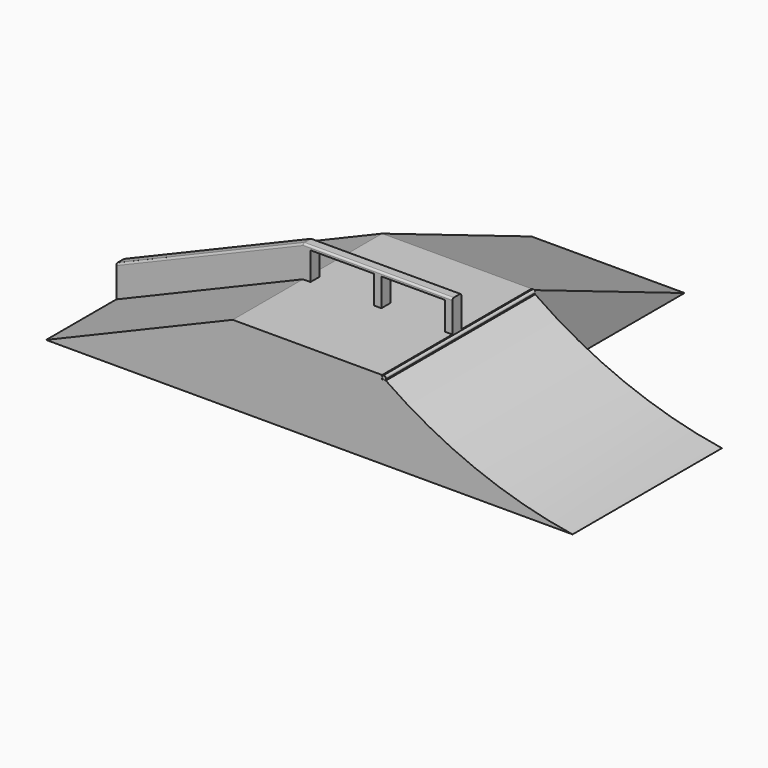
from build123d import *

# Parameters (mm, degrees)
F1_DEPTH     = 127
F2_W         = 5.08
F2_H         = 7.62
F3_DEPTH     = 19.05
F4_W         = 7.62
F4_H         = 2.54
F5_DEPTH     = 101.6
F6_T         = 5.08
F6_T3_DEPTH  = 17.78
F6_T5_DEPTH  = 15.24
F6_T7_DEPTH  = 15.24
F6_T9_DEPTH  = 15.24
F6_T11_DEPTH = 137.16
F8_DEPTH     = 7.62
F10_DEPTH    = 104.14
F11_R        = 1.27


# Not quite as in the source:
# - a shell that OpenCascade refuses in one call is made with other operations: the cavity is built on its own and cut out
# - a feature names something its author has since deleted; it is built from what else it names


with BuildPart() as f1:
    # F0 (on Front) → F1 (new body)
    with BuildSketch(Plane.XZ):
        with BuildLine():
            Line((0, 50.8), (0, 0))
            Line((0, 0), (127, 0))
            ThreePointArc((127, 0), (60.6135499229, 18.1838748072), (0, 50.8))
        make_face()
        Polygon((-104.14, 0), (-2.54, 0), (-2.54, 50.8), (-2.54, 52.07), (-2.54, 53.34), (-104.14, 53.34), align=None)
        Polygon((-2.54, 0), (0, 0), (0, 50.8), (-1.27, 50.8), (-2.54, 50.8), align=None)
        Polygon((-231.14, 0), (-104.14, 0), (-104.14, 53.34), align=None)
    extrude(amount=F1_DEPTH)

    # F2 (on face) → F3 (join)
    with BuildSketch(Plane.XY.offset(53.34)):
        with Locations((-101.6, -63.5)):
            Rectangle(F2_W, F2_H)
        with Locations((-5.08, -63.5)):
            Rectangle(F2_W, F2_H)
        with Locations((-53.34, -63.5)):
            Rectangle(F2_W, F2_H)
    extrude(amount=F3_DEPTH)

    # F4 (on face) → F5 (join)
    with BuildSketch(Plane.YZ.offset(-2.54)):
        with Locations((-63.5, 73.66)):
            Rectangle(F4_W, F4_H)
    extrude(amount=-F5_DEPTH)

    # F6: shell of thickness 5.08, made by hand


with BuildPart() as f1b:
    # F0 (on Front) → F1, piece 2 (new body)
    with BuildSketch(Plane.XZ):
        with BuildLine():
            ThreePointArc((-2.54, 52.07), (-2.1680256121, 51.1719743879), (-1.27, 50.8))
            ThreePointArc((-1.27, 50.8), (-0.3719743879, 51.1719743879), (0, 52.07))
            ThreePointArc((0, 52.07), (-1.27, 53.34), (-2.54, 52.07))
        make_face()
    extrude(amount=F1_DEPTH)


with BuildPart() as f6_core1:
    # F6_t2: copy of F1
    add(f1.part)

    # the walls: a layer under each face that stays
    f6_faces = [f6_core1.faces().sort_by_distance(p)[0] for p in [
        (60.6135499229, -63.5, 18.1838748072),
        (-52.07, -127, 26.67),
        (-167.64, -63.5, 26.67),
        (-104.14, -63.5, 64.135),
        (-53.34, -67.31, 64.135),
        (-99.06, -63.5, 62.865),
        (-77.47, -63.5, 72.39),
        (-55.88, -63.5, 62.865),
        (-50.8, -63.5, 62.865),
        (-29.21, -63.5, 72.39),
        (-7.62, -63.5, 62.865),
        (-53.34, -63.5, 74.93),
        (-53.34, -59.69, 64.135),
        (-19.4733333333, -105.8333333333, 53.34),
        (-2.54, -63.5, 62.865),
        (-52.07, 0, 26.67),
        (-1.27, -63.5, 50.8),
    ]]
    thicken(f6_faces, amount=-F6_T, mode=Mode.SUBTRACT)

    # F6_s4 → F6_t3 (cut)
    with BuildSketch(Plane.XZ.offset(54.61)):
        Polygon((-104.2104714102, 53.386836691), (-102.1728589795, 48.6563309035), (-99.06, 49.9637316749), (-99.06, 53.34), align=None)
        Polygon((-99.0092, 53.3908), (-104.14, 53.34), (-104.14, 48.26), (-99.06, 48.26), align=None)
        Polygon((-99.0092, 72.3392), (-104.14, 72.39), (-104.14, 77.47), (-99.06, 77.47), align=None)
        Polygon((-55.9308, 72.3392), (-55.88, 77.47), (-50.8, 77.47), (-50.8, 72.39), align=None)
        Polygon((-55.9308, 53.3908), (-50.8, 53.34), (-50.8, 48.26), (-55.88, 48.26), align=None)
        Polygon((-50.7492, 53.3908), (-55.88, 53.34), (-55.88, 48.26), (-50.8, 48.26), align=None)
        Polygon((-50.7492, 72.3392), (-55.88, 72.39), (-55.88, 77.47), (-50.8, 77.47), align=None)
        Polygon((-7.6708, 72.3392), (-7.62, 77.47), (-2.54, 77.47), (-2.54, 72.39), align=None)
        Polygon((-7.6708, 53.3908), (-2.54, 53.34), (-2.54, 48.26), (-7.62, 48.26), align=None)
    extrude(amount=F6_T3_DEPTH, mode=Mode.SUBTRACT)

    # F6_s6 → F6_t5 (cut)
    with BuildSketch(Plane.YZ.offset(-60.96)):
        Polygon((-67.3608, 53.3908), (-62.23, 53.34), (-62.23, 48.26), (-67.31, 48.26), align=None)
        Polygon((-59.6392, 53.3908), (-64.77, 53.34), (-64.77, 48.26), (-59.69, 48.26), align=None)
    extrude(amount=F6_T5_DEPTH, mode=Mode.SUBTRACT)

    # F6_s8 → F6_t7 (cut)
    with BuildSketch(Plane.YZ.offset(-109.22)):
        Polygon((-67.3608, 53.3908), (-62.23, 53.34), (-62.23, 48.26), (-67.31, 48.26), align=None)
        Polygon((-59.6392, 53.3908), (-64.77, 53.34), (-64.77, 48.26), (-59.69, 48.26), align=None)
    extrude(amount=F6_T7_DEPTH, mode=Mode.SUBTRACT)

    # F6_s10 → F6_t9 (cut)
    with BuildSketch(Plane.YZ.offset(-12.7)):
        Polygon((-67.3608, 53.3908), (-62.23, 53.34), (-62.23, 48.26), (-67.31, 48.26), align=None)
        Polygon((-59.6392, 53.3908), (-64.77, 53.34), (-64.77, 48.26), (-59.69, 48.26), align=None)
    extrude(amount=F6_T9_DEPTH, mode=Mode.SUBTRACT)

    # F6_s12 → F6_t11 (cut)
    with BuildSketch(Plane.XZ.offset(-5.08)):
        Polygon((-2.4892, 50.8508), (-7.62, 50.8), (-7.62, 45.72), (-2.54, 45.72), align=None)
    extrude(amount=F6_T11_DEPTH, mode=Mode.SUBTRACT)


with BuildPart() as f1_1:
    add(f1.part)

    # what is left inside the walls is the cavity
    f6_cavity = [f6_core1.part.solids().sort_by_distance(p)[0] for p in [
        (-58.552758, -82.973333, 0.0508),
    ]]
    add(f6_cavity, mode=Mode.SUBTRACT)

    # F7 (on face) → F8 (join)
    with BuildSketch(Plane(origin=(0, -59.69, 0), x_dir=(-1, 0, 0), z_dir=(0, 1, 0))):
        Polygon((231.14, 21.59), (104.14, 74.93), (104.14, 53.34), (231.14, 0), align=None)
    extrude(amount=-F8_DEPTH)

    # F9 (on Right) → F10 (join)
    with BuildSketch(Plane.YZ):
        Polygon((127, 0), (0, 53.34), (0, 0), align=None)
    extrude(amount=-F10_DEPTH)

    # F11
    f11_edges = [f1_1.edges().sort_by_distance(p)[0] for p in [
        (-53.34, -67.31, 74.93),
        (-167.64, -67.31, 48.26),
        (-104.14, -63.5, 74.93),
        (-167.64, -59.69, 48.26),
        (-53.34, -59.69, 74.93),
    ]]
    fillet(f11_edges, radius=F11_R)


solid = Compound([f1b.part, f1_1.part])
